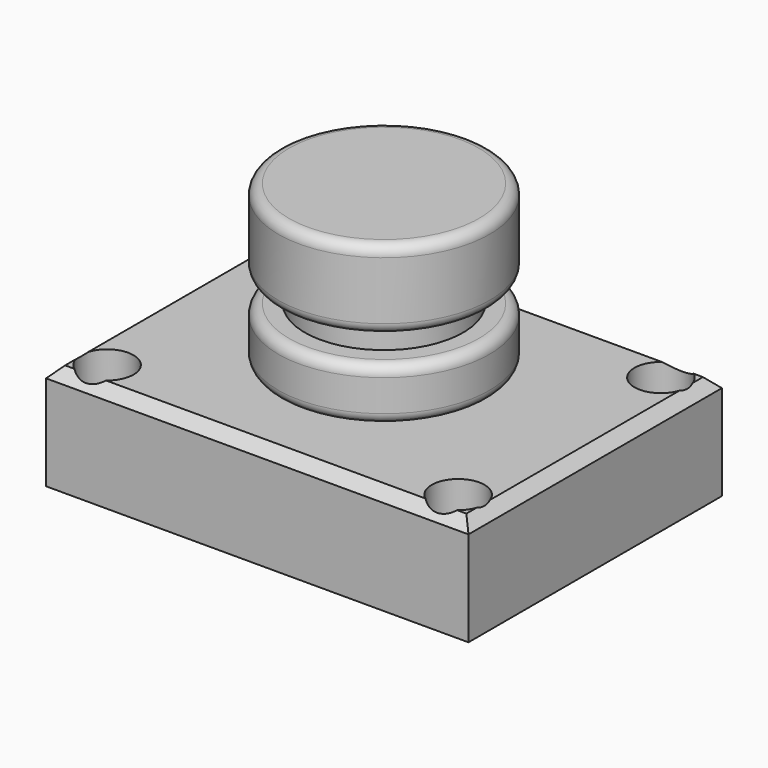
from build123d import *

# Parameters (mm, degrees)
F0_W        = 101.6
F0_H        = 76.2
F1_DEPTH    = 25.4
F2_R        = 6.35
F3_DEPTH    = 25.4
F4_W        = 25.4
F4_H        = 38.1
F6_W        = 23.2788839974
F6_H        = 6.35
F8_T1_DEPTH = 114.6641495789
F8_T3_DEPTH = 89.2641495789
F9_R        = 2.54


# Not quite as in the source:
# - a fillet or chamfer that OpenCascade refuses, or shapes differently, is made with other operations: its cross-section is extruded or revolved along the edge and cut away or added
# - a feature names something its author has since deleted; it is built from what else it names


with BuildPart() as f1:
    # F0 (on Top) → F1 (new body)
    with BuildSketch(Plane.XY):
        Rectangle(F0_W, F0_H)
    extrude(amount=F1_DEPTH)

    # F2 (on face) → F3 (cut)
    with BuildSketch(Plane(origin=(0, 0, 0), x_dir=(1, 0, 0), z_dir=(0, 0, -1))):
        with Locations((-42.2228313982, -30.48)):
            Circle(F2_R)
        with Locations((-42.2228313982, 30.48)):
            Circle(F2_R)
        with Locations((42.2228313982, 30.48)):
            Circle(F2_R)
        with Locations((42.2228313982, -30.48)):
            Circle(F2_R)
    extrude(amount=-F3_DEPTH, mode=Mode.SUBTRACT)

    # F8: chamfer of 2.54 on 4 edges, made by hand

    # F8_s2 → F8_t1 (cut)
    with BuildSketch(Plane.YZ.offset(-57.3320747894)):
        Polygon((-38.1, 22.86), (-35.56, 25.4), (-38.1, 25.4), align=None)
        Polygon((38.1, 22.86), (35.56, 25.4), (38.1, 25.4), align=None)
    extrude(amount=F8_T1_DEPTH, mode=Mode.SUBTRACT)

    # F8_s4 → F8_t3 (cut)
    with BuildSketch(Plane.XZ.offset(-44.6320747894)):
        Polygon((50.8, 22.86), (48.26, 25.4), (50.8, 25.4), align=None)
        Polygon((-48.26, 25.4), (-50.8, 22.86), (-50.8, 25.4), align=None)
    extrude(amount=F8_T3_DEPTH, mode=Mode.SUBTRACT)


with BuildPart() as f5:
    # F4 (on Front) → F5 (revolve)
    with BuildSketch(Plane.XZ):
        with Locations((-12.7, 46.1308773281)):
            Rectangle(F4_W, F4_H)
    revolve(axis=Axis((0, 0, 46.1308773281), (0, 0, 1)))

    # F6 (on Right) → F7 (revolve, cut)
    with BuildSketch(Plane.YZ):
        with Locations((-30.6894419987, 42.9558773281)):
            Rectangle(F6_W, F6_H)
    revolve(axis=Axis((0, 0, 65.1808773281), (0, 0, -1)), mode=Mode.SUBTRACT)

    # F9
    f9_edges = [f5.edges().sort_by_distance(p)[0] for p in [
        (25.4, 0, 27.080877),
        (25.4, 0, 39.780877),
        (25.4, 0, 46.130877),
        (25.4, 0, 65.180877),
    ]]
    fillet(f9_edges, radius=F9_R)


solid = Compound([f1.part, f5.part])
